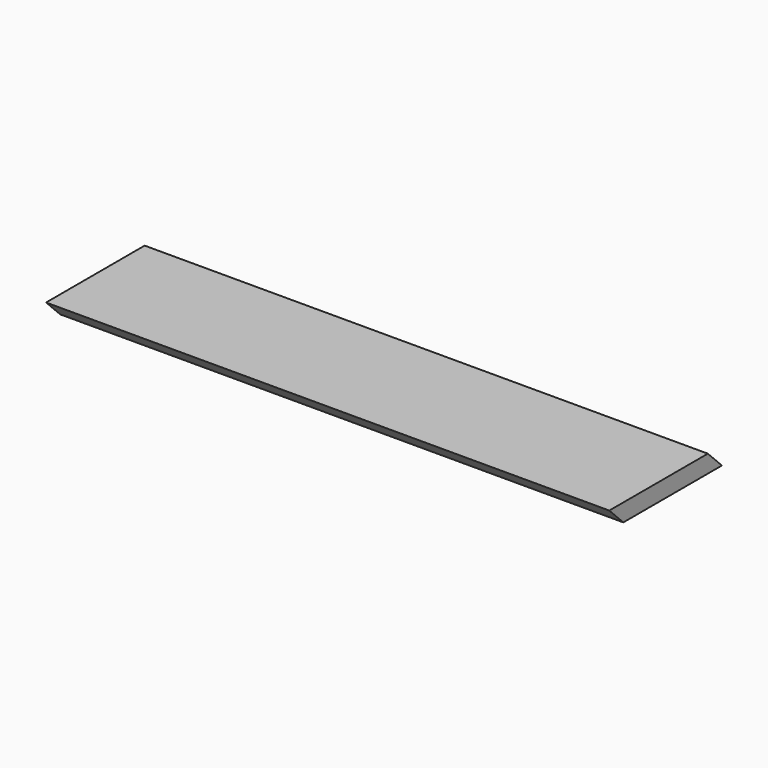
from build123d import *

# Parameters (mm, degrees)
F0_W     = 101.6
F0_H     = 25.4
F1_DEPTH = 3.175
F2_SIZE  = 3.17499
F3_SIZE  = 3.17499


# Not quite as in the source:
# - a fillet or chamfer is up to 0.001 mm smaller than in the source, because OpenCascade refuses the exact size
# - a length typed as a fraction of an inch, garbled in the dataset ("3 / 203.2 mm" for 3/8 in), is restored


with BuildPart() as f1:
    # F0 (on Top) → F1 (new body)
    with BuildSketch(Plane.XY):
        Rectangle(F0_W, F0_H)
    extrude(amount=F1_DEPTH)

    # F2 (size 3.175 in the source; OpenCascade refuses exactly that, so slightly less here)
    f2_edges = [f1.edges().sort_by_distance(p)[0] for p in [
        (0, 12.7, 3.175),
    ]]
    chamfer(f2_edges, length=F2_SIZE)

    # F3 (size 3.175 in the source; OpenCascade refuses exactly that, so slightly less here)
    f3_edges = [f1.edges().sort_by_distance(p)[0] for p in [
        (0, -12.7, 0),
    ]]
    chamfer(f3_edges, length=F3_SIZE)


solid = f1.part
